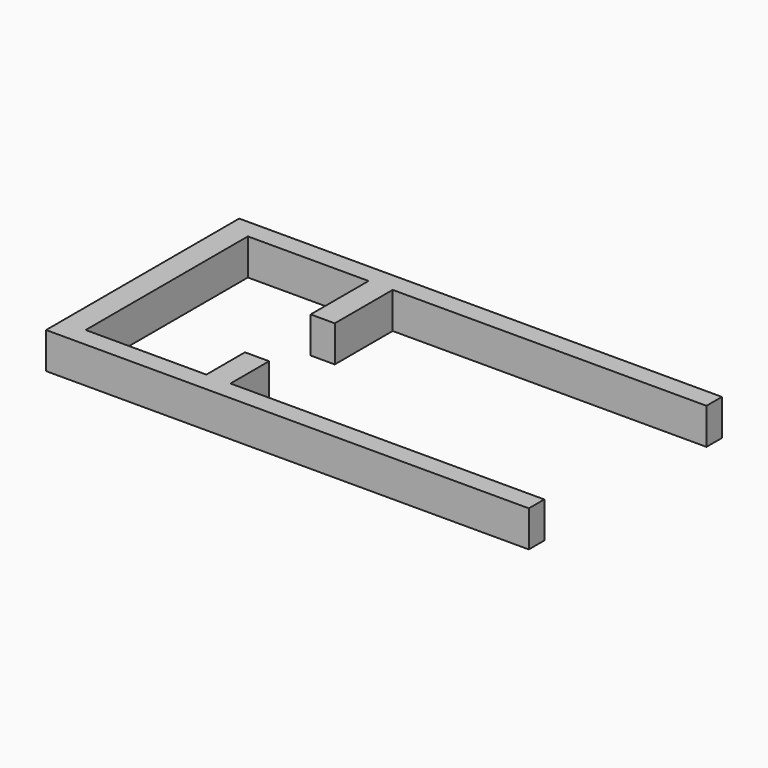
from build123d import *

# Parameters (mm, degrees)
F1_DEPTH = 15


# Not quite as in the source:
# - a feature names something its author has since deleted; it is built from what else it names


with BuildPart() as f1:
    # F0 (on Top) → F1 (new body)
    with BuildSketch(Plane.XY):
        Polygon((-100, -50), (100, -50), (100, -42), (-30, -42), (-30, -22), (-40, -22), (-40, -42), (-90, -42), (-90, 42), (-40, 42), (-40, 12), (-30, 12), (-30, 42), (-6.4, 42), (100, 42), (100, 50), (-100, 50), align=None)
    extrude(amount=F1_DEPTH)


solid = f1.part
